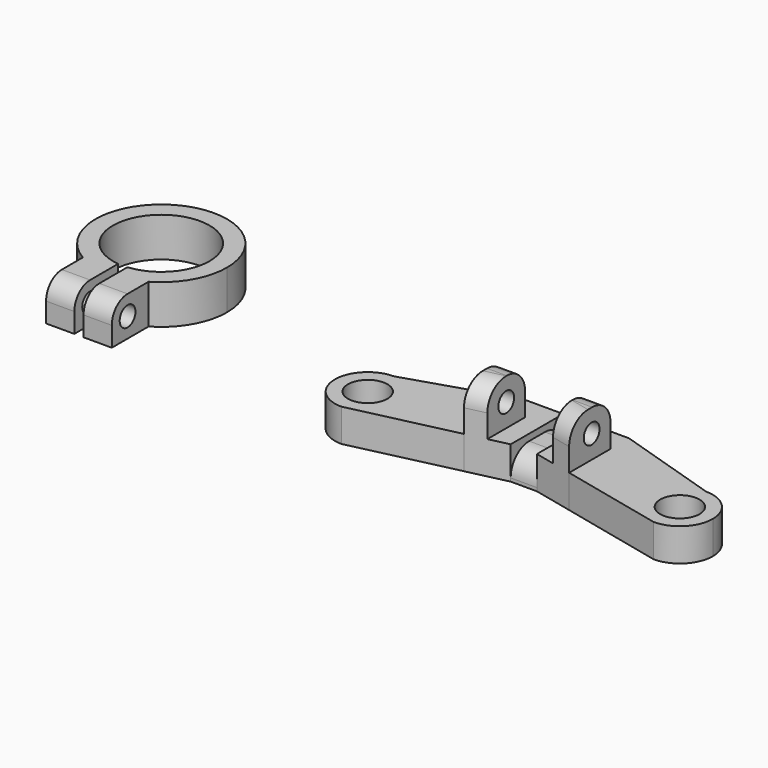
from build123d import *

# Parameters (mm, degrees)
F1_DEPTH = 6
F3_D     = 3
F5_DEPTH = 12
F4_R     = 3
F4_W     = 3
F4_H     = 3.5
F6_DEPTH = 5
F4_W_2   = 2
F4_H_2   = 10
F7_DEPTH = 4
F8_R     = 4.99999
F9_R     = 3.5
F11_D    = 3
F13_R    = 3


# Not quite as in the source:
# - a fillet or chamfer is up to 0.001 mm smaller than in the source, because OpenCascade refuses the exact size
# - a feature names something its author has since deleted; it is built from what else it names


with BuildPart() as f1:
    # F0 (on Top) → F1 (new body)
    with BuildSketch(Plane.XY):
        with BuildLine():
            ThreePointArc((-26.4478022211, 9.2937625569), (-28.5229179157, 8.3913259797), (-30.7478022211, 7.978546681))
            Line((-30.7478022211, 7.978546681), (-30.7478022211, 2.2937625569))
            Line((-30.7478022211, 2.2937625569), (-26.4478022211, 2.2937625569))
            Line((-26.4478022211, 2.2937625569), (-26.4478022211, 9.2937625569))
        make_face()
        with BuildLine():
            Line((-32.1478022211, 2.2937625569), (-32.1478022211, 7.978546681))
            ThreePointArc((-32.1478022211, 7.978546681), (-34.3726865265, 8.3913259797), (-36.4478022211, 9.2937625569))
            Line((-36.4478022211, 9.2937625569), (-36.4478022211, 2.2937625569))
            Line((-36.4478022211, 2.2937625569), (-32.1478022211, 2.2937625569))
        make_face()
        with BuildLine():
            ThreePointArc((-32.1478022211, 10.6374258586), (-36.3913586332, 23.3931111885), (-24.0978022211, 17.9540165948))
            ThreePointArc((-24.0978022211, 17.9540165948), (-26.0087076273, 13.0104601826), (-30.7478022211, 10.6374258586))
            Line((-30.7478022211, 10.6374258586), (-30.7478022211, 7.978546681))
            ThreePointArc((-30.7478022211, 7.978546681), (-28.5229179157, 8.3913259797), (-26.4478022211, 9.2937625569))
            ThreePointArc((-26.4478022211, 9.2937625569), (-22.7875481833, 12.9540165948), (-21.4478022211, 17.9540165948))
            ThreePointArc((-21.4478022211, 17.9540165948), (-36.4478022211, 26.6142706326), (-36.4478022211, 9.2937625569))
            ThreePointArc((-36.4478022211, 9.2937625569), (-34.3726865265, 8.3913259797), (-32.1478022211, 7.978546681))
            Line((-32.1478022211, 7.978546681), (-32.1478022211, 10.6374258586))
        make_face()
    extrude(amount=F1_DEPTH)

    # F3 (through all)
    with Locations(Plane.YZ.offset(-26.4478022211)):
        with Locations((5.2937625569, 3)):
            Hole(F3_D / 2)

    # F13
    f13_edges = [f1.edges().sort_by_distance(p)[0] for p in [
        (-34.297802, 2.293763, 6),
        (-28.597802, 2.293763, 6),
    ]]
    fillet(f13_edges, radius=F13_R)


with BuildPart() as f5:
    # F4 (on Top) → F5 (new body)
    with BuildSketch(Plane.XY):
        Polygon((26.0828619152, 5), (26.0828619152, 3.6206896552), (29.0828619152, 4.3103448276), (29.0828619152, 5), (29.0828619152, 11.5), (26.0828619152, 11.5), align=None)
    extrude(amount=F5_DEPTH)

    # F4 (on Top) → F6 (join)
    with BuildSketch(Plane.XY):
        Polygon((10.3328619152, 10), (5.3328619152, 10), (5.3328619152, 0), (10.3328619152, 0), (26.0828619152, 3.6206896552), (26.0828619152, 5), (26.0828619152, 11.5), (26.0828619152, 15), align=None)
        with Locations((10.3328619152, 5)):
            Circle(F4_R, mode=Mode.SUBTRACT)
        Polygon((32.0828619152, 15), (29.0828619152, 15), (29.0828619152, 11.5), (29.0828619152, 5), (29.0828619152, 4.3103448276), (32.0828619152, 5), align=None)
        with Locations((27.5828619152, 13.25)):
            Rectangle(F4_W, F4_H)
    extrude(amount=F6_DEPTH)

    # F4 (on Top) → F7 (join)
    with BuildSketch(Plane.XY):
        with Locations((33.0828619152, 10)):
            Rectangle(F4_W_2, F4_H_2)
    extrude(amount=F7_DEPTH)

    # F8 (radius 5 in the source; OpenCascade refuses exactly that, so slightly less here)
    f8_edges = [f5.edges().sort_by_distance(p)[0] for p in [
        (5.332862, 0, 2.5),
        (5.332862, 10, 2.5),
    ]]
    fillet(f8_edges, radius=F8_R)

    # F9
    f9_edges = [f5.edges().sort_by_distance(p)[0] for p in [
        (33.082862, 15, 4),
        (33.082862, 5, 4),
        (27.582862, 11.5, 12),
        (27.582862, 3.965517, 12),
    ]]
    fillet(f9_edges, radius=F9_R)

    # F11 (through all)
    with Locations(Plane.YZ.offset(29.0828619152)):
        with Locations((7.9016367206, 8.5)):
            Hole(F11_D / 2)

    # F12: F5 across face


with BuildPart() as f5_1:
    add(f5.part)
    add(f5.part.mirror(Plane(origin=(34.0828619152, 10, 1.8156409487), x_dir=(0, 1, 0), z_dir=(1, 0, 0))))


solid = Compound([f1.part, f5_1.part])
